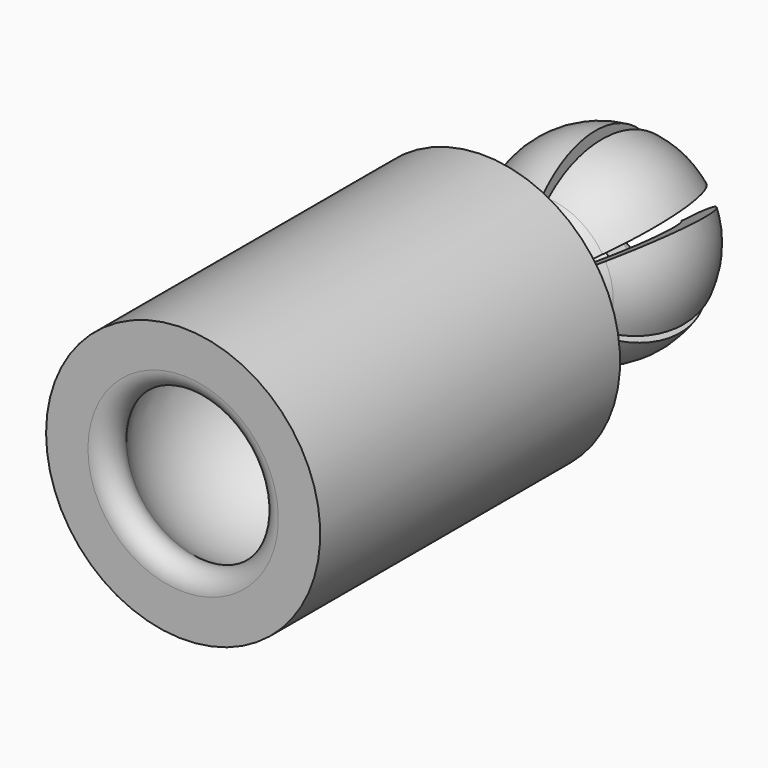
from build123d import *

# Parameters (mm, degrees)
F2_R            = 0.3
F4_W            = 0.8
F4_H            = 10
F5_DEPTH        = 7
F5_TAPER        = 3
F5_COPIES_COUNT = 3
F5_COPIES_ANGLE = 120


# Not quite as in the source:
# - a pattern or mirror of a feature is missing from the dataset's text; its kind, count and spacing are read off the source's solid


with BuildPart() as f1:
    # F0 (on Top) → F1 (revolve)
    with BuildSketch(Plane.XY):
        with BuildLine():
            Line((-3.6616241559, 18.1017866649), (-5, 18.1017866649))
            Line((-5, 18.1017866649), (-5, 4.4295576802))
            Line((-5, 4.4295576802), (-3.4733384694, 4.4295576802))
            ThreePointArc((-3.4733384694, 4.4295576802), (-2.858229425, 4.8289882129), (-2.9728969919, 5.5533881273))
            ThreePointArc((-2.9728969919, 5.5533881273), (-3.6540852625, 9.8567211306), (0, 12.2295576802))
            Line((0, 12.2295576802), (0, 13.2295576802))
            Line((0, 13.2295576802), (-1.75, 13.2295576802))
            ThreePointArc((-1.75, 13.2295576802), (-2.8106601718, 13.6688975084), (-3.25, 14.7295576802))
            Line((-3.25, 14.7295576802), (-3.25, 15.133903629))
            ThreePointArc((-3.25, 15.133903629), (-2.9180360672, 16.3669647589), (-2.0118819111, 17.2667005246))
            ThreePointArc((-2.0118819111, 17.2667005246), (-1.1950672071, 18.0174138879), (-0.7848536925, 19.0481814112))
            ThreePointArc((-0.7848536925, 19.0481814112), (-0.9082840984, 20.4490964914), (-1.6699842869, 21.631302459))
            ThreePointArc((-1.6699842869, 21.631302459), (-2.4331664821, 23.3455486703), (-1.75, 25.093224468))
            Line((-1.75, 25.093224468), (-1.75, 26.4332006489))
            ThreePointArc((-1.75, 26.4332006489), (-3.4695934856, 23.8642710291), (-2.4829425749, 20.93460874))
            ThreePointArc((-2.4829425749, 20.93460874), (-2.1274980872, 19.1250911197), (-3.6616241559, 18.1017866649))
        make_face()
    revolve(axis=Axis((0, 19.0359335393, 0), (0, 1, 0)))

    # F2
    f2_edges = [f1.edges().sort_by_distance(p)[0] for p in [
        (1.75, 26.433201, 0),
    ]]
    fillet(f2_edges, radius=F2_R)

    # F4 (on offset) → F5 (cut)
    with BuildSketch(Plane.XZ.offset(-26.5)):
        Rectangle(F4_W, F4_H)
    f5 = extrude(amount=F5_DEPTH, taper=F5_TAPER, mode=Mode.SUBTRACT)

    # F5_copies: F5 ×3 about axis
    f5_copies_axis = Axis((0, 0, 0), (0, 1, 0))
    for i in range(1, F5_COPIES_COUNT):
        add(f5.rotate(f5_copies_axis, i * F5_COPIES_ANGLE / (F5_COPIES_COUNT - 1)), mode=Mode.SUBTRACT)


solid = f1.part
